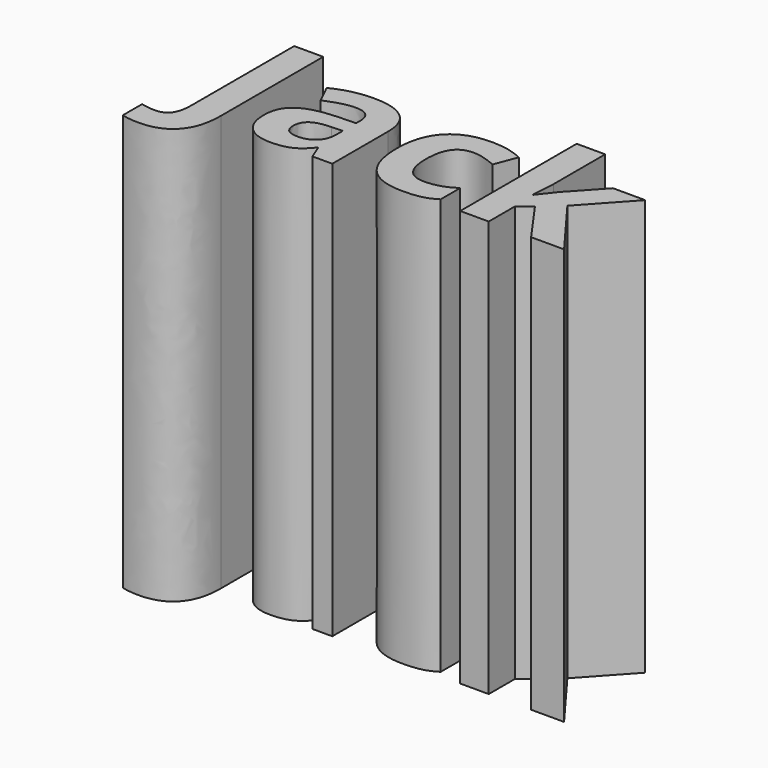
from build123d import *

# Parameters (mm, degrees)
F0_TEXT_SIZE = 11.6973691749
F1_DEPTH     = 25.4


# Not quite as in the source:
# - Text() gives the source's letters only with a copy of the font that has no kerning and outlines rounded to 1/6400 em; it was checked with that copy


with BuildPart() as f1:
    # F0 (on Top) → F1 (new body)
    with BuildSketch(Plane.XY):
        with Locations((-23.0103954673, -5.8653950691)):
            Text('Jack', F0_TEXT_SIZE, font='Open Sans', font_style=FontStyle.BOLD, text_align=(TextAlign.LEFT, TextAlign.BOTTOM))
    extrude(amount=F1_DEPTH)


solid = f1.part
